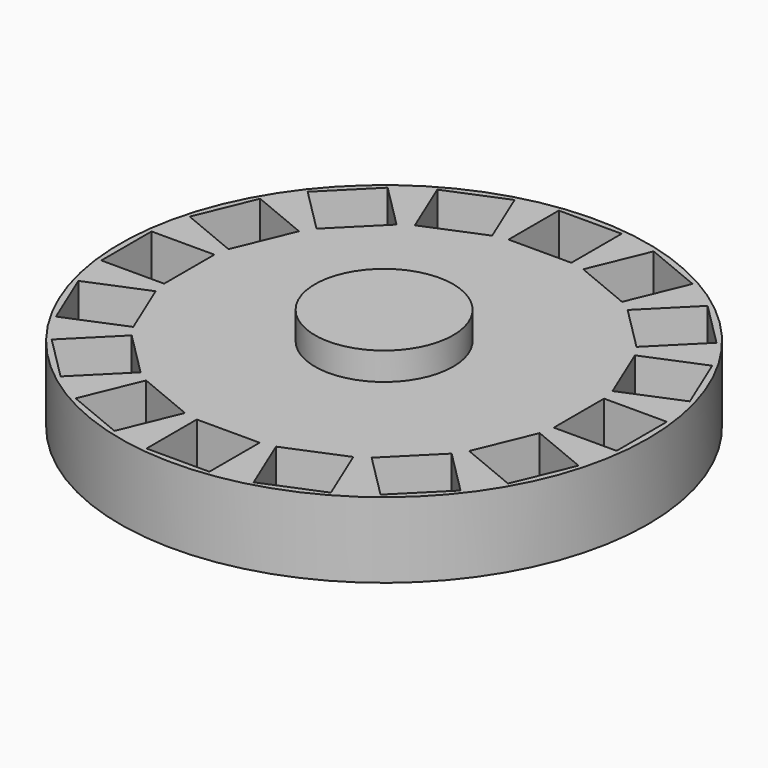
from build123d import *

# Parameters (mm, degrees)
F0_W     = 21
F0_H     = 6
F2_R     = 5
F3_DEPTH = 25
F4_W     = 5
F4_H     = 5
F5_DEPTH = 5
F2_R_2   = 5.5
F6_DEPTH = 8.2


# Not quite as in the source:
# - a feature names something its author has since deleted; it is built from what else it names


with BuildPart() as f1:
    # F0 (on Front) → F1 (revolve)
    with BuildSketch(Plane.XZ):
        with Locations((10.5, 3)):
            Rectangle(F0_W, F0_H)
    revolve(axis=Axis((0, 0, 3), (0, 0, -1)))

    # F2 (on Top) → F3 (cut)
    with BuildSketch(Plane.XY):
        Circle(F2_R)
    extrude(amount=F3_DEPTH, mode=Mode.SUBTRACT)

    # F4 (on face) → F5 (cut)
    with BuildSketch(Plane.XY.offset(6)):
        with Locations((0, 18)):
            Rectangle(F4_W, F4_H)
        Polygon((5.5353115322, 19.8962389974), (3.6218943704, 15.2768413348), (8.2412920329, 13.363424173), (10.1547091948, 17.9828218356), align=None)
        Polygon((12.7279220614, 16.2634559673), (9.1923881554, 12.7279220614), (12.7279220614, 9.1923881554), (16.2634559673, 12.7279220614), align=None)
        Polygon((17.9828218356, 10.1547091948), (13.363424173, 8.2412920329), (15.2768413348, 3.6218943704), (19.8962389974, 5.5353115322), align=None)
        with Locations((18, 0)):
            Rectangle(F4_W, F4_H)
        Polygon((19.8962389974, -5.5353115322), (15.2768413348, -3.6218943704), (13.363424173, -8.2412920329), (17.9828218356, -10.1547091948), align=None)
        Polygon((16.2634559673, -12.7279220614), (12.7279220614, -9.1923881554), (9.1923881554, -12.7279220614), (12.7279220614, -16.2634559673), align=None)
        Polygon((10.1547091948, -17.9828218356), (8.2412920329, -13.363424173), (3.6218943704, -15.2768413348), (5.5353115322, -19.8962389974), align=None)
        with Locations((0, -18)):
            Rectangle(F4_W, F4_H)
        Polygon((-5.5353115322, -19.8962389974), (-3.6218943704, -15.2768413348), (-8.2412920329, -13.363424173), (-10.1547091948, -17.9828218356), align=None)
        Polygon((-12.7279220614, -16.2634559673), (-9.1923881554, -12.7279220614), (-12.7279220614, -9.1923881554), (-16.2634559673, -12.7279220614), align=None)
        Polygon((-17.9828218356, -10.1547091948), (-13.363424173, -8.2412920329), (-15.2768413348, -3.6218943704), (-19.8962389974, -5.5353115322), align=None)
        with Locations((-18, 0)):
            Rectangle(F4_W, F4_H)
        Polygon((-19.8962389974, 5.5353115322), (-15.2768413348, 3.6218943704), (-13.363424173, 8.2412920329), (-17.9828218356, 10.1547091948), align=None)
        Polygon((-16.2634559673, 12.7279220614), (-12.7279220614, 9.1923881554), (-9.1923881554, 12.7279220614), (-12.7279220614, 16.2634559673), align=None)
        Polygon((-10.1547091948, 17.9828218356), (-8.2412920329, 13.363424173), (-3.6218943704, 15.2768413348), (-5.5353115322, 19.8962389974), align=None)
    extrude(amount=-F5_DEPTH, mode=Mode.SUBTRACT)

    # F2 (on Top) → F6 (join)
    with BuildSketch(Plane.XY):
        Circle(F2_R_2)
        Circle(F2_R, mode=Mode.SUBTRACT)
    extrude(amount=F6_DEPTH)

    # F7 (on Right) → F8 (revolve)
    with BuildSketch(Plane.YZ):
        Polygon((0, 8.2), (0, 8), (5.5, 8), (5.5, 8.2), (5.4786731489, 8.2), align=None)
    revolve(axis=Axis((0, 0, 8.1), (0, 0, -1)))


solid = f1.part
